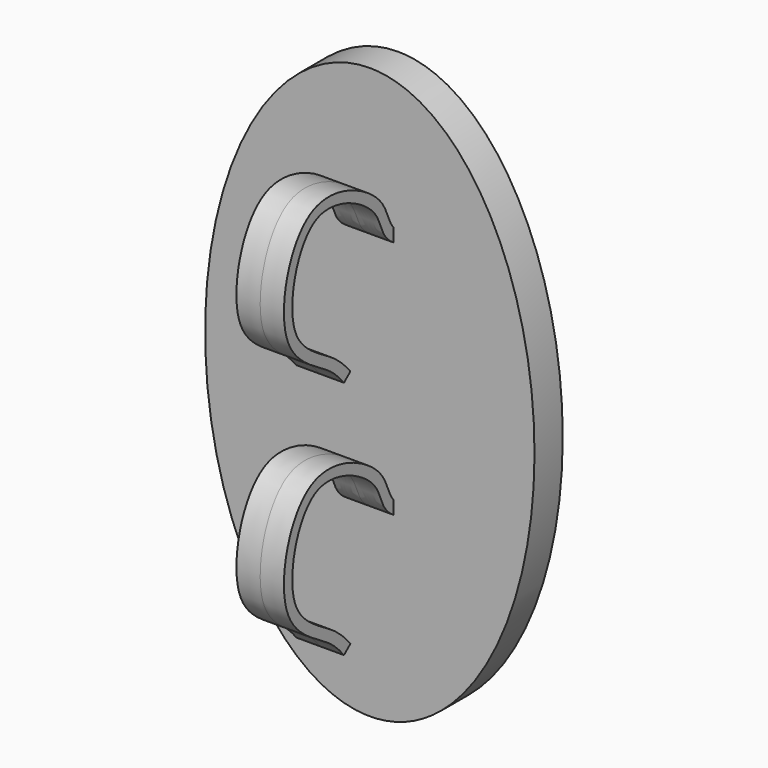
from build123d import *

# Parameters (mm, degrees)
F1_DEPTH = 7.62
F3_DEPTH = 5.1308


# Not quite as in the source:
# - the dataset's text gives a spline's control points without its knots; the knots are read off the source's solid


with BuildPart() as f1:
    # F0 (on Front) → F1 (new body)
    with BuildSketch(Plane.XZ):
        with BuildLine():
            add(Edge.make_bspline(
                [(0, 61.6552382708), (-61.6231878011, 61.6552382708), (-30.8115939005, -30.8276191354), (0, -123.3104765415), (30.8115939005, -30.8276191354), (61.6231878011, 61.6552382708), (0, 61.6552382708)],
                knots=[0, 0, 0, 2.0943951024, 2.0943951024, 4.1887902048, 4.1887902048, 6.2831853072, 6.2831853072, 6.2831853072], degree=2, weights=[1, 0.5, 1, 0.5, 1, 0.5, 1]))
        make_face()
    extrude(amount=F1_DEPTH)

    # F2 (on Right) → F3 (join, symmetric)
    with BuildSketch(Plane.YZ):
        with BuildLine():
            Line((-0.975969542, -24.6715213086), (-0.0573207641, -22.6059956476))
            add(Edge.make_bspline(
                [(-0.0573207641, -22.6059956476), (-3.0870333212, -21.2585218349), (-9.0815402196, -19.5987906342), (-9.1994884916, -11.0204376563), (-33.1797326707, 0.8717861567), (-41.2298457398, -31.1634849674), (-25.1331714992, -38.0243579735), (-22.1681455361, -41.5290663185), (-21.009165516, -42.8998032585)],
                knots=[0, 0, 0, 0, 0.1391479132, 0.2671564695, 0.47352574, 0.7001382698, 0.8833436719, 1, 1, 1, 1], degree=3))
            Line((-21.009165516, -42.8998032585), (-19.2829117425, -41.4402280659))
            add(Edge.make_bspline(
                [(-0.975969542, -24.6715213086), (-1.6117193564, -24.388769658), (-2.9299369677, -23.8524399416), (-4.6050999175, -23.1892244992), (-5.9177080285, -22.6060074903), (-6.8797496614, -22.1222840405), (-7.6554550512, -21.6597734273), (-8.2539426636, -21.2374146947), (-8.6889362559, -20.889592338), (-9.0368557663, -20.5694408932), (-9.3032721054, -20.2933503161), (-9.5618768934, -20.0014857224), (-9.8515717918, -19.6278491535), (-10.2491256448, -19.0250203377), (-10.6387010555, -18.2829201929), (-10.9998789752, -17.444162587), (-11.3134926587, -16.6605001008), (-11.6239768052, -15.9239172057), (-11.9671940183, -15.2203138176), (-12.3089995451, -14.6456797706), (-12.6363664777, -14.1818297468), (-12.913813658, -13.8304030687), (-13.2330879472, -13.4693770813), (-13.7268592946, -12.9651872945), (-14.456201062, -12.3139086955), (-15.4848337669, -11.5319242687), (-16.638662136, -10.7786420211), (-18.307916831, -9.8454388054), (-20.5722110312, -8.8694956097), (-22.888681573, -8.2812166075), (-24.6573350622, -8.1022585071), (-25.9138338198, -8.1218738499), (-27.0765700191, -8.2987936017), (-27.9584843365, -8.5780944086), (-28.6092112644, -8.8813615598), (-29.2503703846, -9.2518975274), (-30.034268134, -9.8423225839), (-30.9352923343, -10.7507776494), (-32.0601124534, -12.2083209675), (-33.2782554898, -14.4362472908), (-34.335682216, -17.5327999172), (-34.9262918503, -20.806795789), (-34.9982826252, -23.4744926574), (-34.8001110398, -25.4428036305), (-34.5730287745, -26.5756949802), (-34.333119555, -27.4085495205), (-34.0576798159, -28.1836758637), (-33.4700300657, -29.4380035427), (-32.3537826425, -31.0042109156), (-30.644012928, -32.6292228307), (-28.6829733473, -34.0490374065), (-26.9676929478, -35.1072177288), (-25.6212068592, -35.9226488421), (-24.6414388255, -36.5324493982), (-23.699825173, -37.1692312043), (-22.8595144256, -37.8063757241), (-22.1042861182, -38.4418776288), (-21.200698425, -39.2821701698), (-20.2403432245, -40.3070287581), (-19.5934553494, -41.0729451222), (-19.2829117425, -41.4402280659)],
                knots=[0, 0, 0, 0, 0.03125, 0.0625, 0.078125, 0.09375, 0.109375, 0.1171875, 0.125, 0.1328125, 0.13671875, 0.140625, 0.1484375, 0.15625, 0.171875, 0.1875, 0.203125, 0.21875, 0.234375, 0.25, 0.2578125, 0.265625, 0.2734375, 0.28125, 0.296875, 0.3125, 0.328125, 0.34375, 0.375, 0.40625, 0.421875, 0.4375, 0.453125, 0.46875, 0.4765625, 0.484375, 0.5, 0.515625, 0.53125, 0.5625, 0.59375, 0.625, 0.65625, 0.671875, 0.6875, 0.6953125, 0.703125, 0.71875, 0.75, 0.78125, 0.8125, 0.84375, 0.859375, 0.875, 0.890625, 0.90625, 0.921875, 0.9375, 0.96875, 1, 1, 1, 1], degree=3))
        make_face()
        with BuildLine():
            Line((-0.975969542, 27.1256190811), (-0.0573207641, 29.1911447421))
            add(Edge.make_bspline(
                [(-0.0573207641, 29.1911447421), (-3.0870333212, 30.5386185548), (-9.0815402196, 32.1983497554), (-9.1994884916, 40.7767027334), (-33.1797326707, 52.6689265464), (-41.2298457398, 20.6336554223), (-25.1331714992, 13.7727824162), (-22.1681455361, 10.2680740712), (-21.009165516, 8.8973371312)],
                knots=[0, 0, 0, 0, 0.1391479132, 0.2671564695, 0.47352574, 0.7001382698, 0.8833436719, 1, 1, 1, 1], degree=3))
            Line((-21.009165516, 8.8973371312), (-19.2829117425, 10.3569123238))
            add(Edge.make_bspline(
                [(-0.975969542, 27.1256190811), (-1.6117193564, 27.4083707317), (-2.9299369677, 27.9447004481), (-4.6050999175, 28.6079158905), (-5.9177080285, 29.1911328994), (-6.8797496614, 29.6748563492), (-7.6554550512, 30.1373669624), (-8.2539426636, 30.559725695), (-8.6889362559, 30.9075480517), (-9.0368557663, 31.2276994964), (-9.3032721054, 31.5037900736), (-9.5618768934, 31.7956546673), (-9.8515717918, 32.1692912361), (-10.2491256448, 32.7721200519), (-10.6387010555, 33.5142201968), (-10.9998789752, 34.3529778027), (-11.3134926587, 35.1366402889), (-11.6239768052, 35.873223184), (-11.9671940183, 36.5768265721), (-12.3089995451, 37.1514606191), (-12.6363664777, 37.6153106429), (-12.913813658, 37.966737321), (-13.2330879472, 38.3277633083), (-13.7268592946, 38.8319530952), (-14.456201062, 39.4832316942), (-15.4848337669, 40.265216121), (-16.638662136, 41.0184983686), (-18.307916831, 41.9517015843), (-20.5722110312, 42.9276447799), (-22.888681573, 43.5159237821), (-24.6573350622, 43.6948818826), (-25.9138338198, 43.6752665398), (-27.0765700191, 43.498346788), (-27.9584843365, 43.2190459811), (-28.6092112644, 42.9157788299), (-29.2503703846, 42.5452428623), (-30.034268134, 41.9548178058), (-30.9352923343, 41.0463627403), (-32.0601124534, 39.5888194221), (-33.2782554898, 37.3608930989), (-34.335682216, 34.2643404725), (-34.9262918503, 30.9903446007), (-34.9982826252, 28.3226477323), (-34.8001110398, 26.3543367591), (-34.5730287745, 25.2214454095), (-34.333119555, 24.3885908692), (-34.0576798159, 23.613464526), (-33.4700300657, 22.359136847), (-32.3537826425, 20.7929294741), (-30.644012928, 19.167917559), (-28.6829733473, 17.7481029832), (-26.9676929478, 16.6899226609), (-25.6212068592, 15.8744915476), (-24.6414388255, 15.2646909915), (-23.699825173, 14.6279091854), (-22.8595144256, 13.9907646656), (-22.1042861182, 13.3552627609), (-21.200698425, 12.5149702199), (-20.2403432245, 11.4901116315), (-19.5934553494, 10.7241952675), (-19.2829117425, 10.3569123238)],
                knots=[0, 0, 0, 0, 0.03125, 0.0625, 0.078125, 0.09375, 0.109375, 0.1171875, 0.125, 0.1328125, 0.13671875, 0.140625, 0.1484375, 0.15625, 0.171875, 0.1875, 0.203125, 0.21875, 0.234375, 0.25, 0.2578125, 0.265625, 0.2734375, 0.28125, 0.296875, 0.3125, 0.328125, 0.34375, 0.375, 0.40625, 0.421875, 0.4375, 0.453125, 0.46875, 0.4765625, 0.484375, 0.5, 0.515625, 0.53125, 0.5625, 0.59375, 0.625, 0.65625, 0.671875, 0.6875, 0.6953125, 0.703125, 0.71875, 0.75, 0.78125, 0.8125, 0.84375, 0.859375, 0.875, 0.890625, 0.90625, 0.921875, 0.9375, 0.96875, 1, 1, 1, 1], degree=3))
        make_face()
    extrude(amount=F3_DEPTH, both=True)


solid = f1.part
